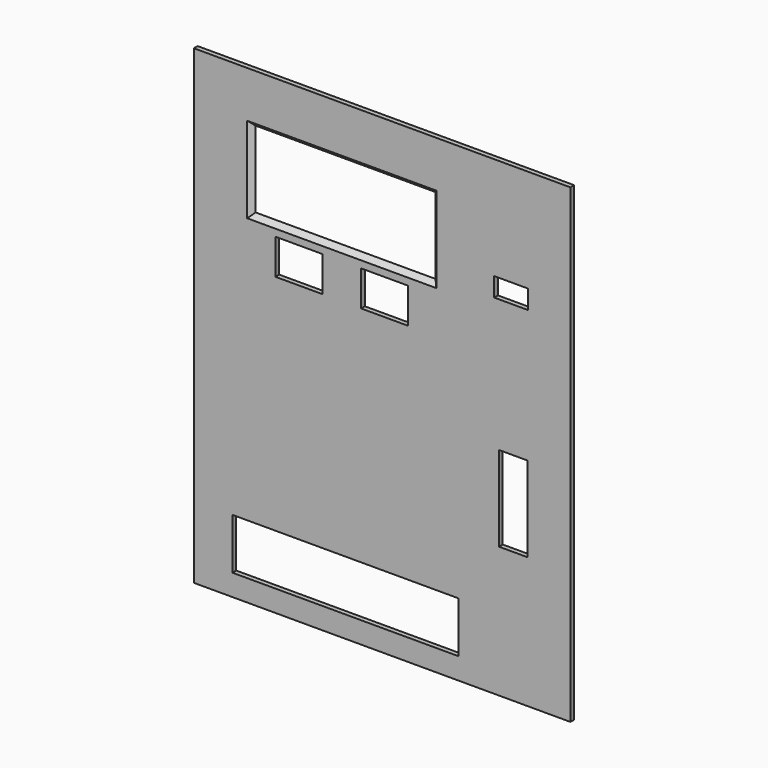
from build123d import *

# Parameters (mm, degrees)
F0_W     = 406.4
F0_H     = 508
F0_W_2   = 244.0329119563
F0_H_2   = 54.9797415733
F0_W_3   = 30.9118032455
F0_H_3   = 91.8955244124
F0_W_4   = 50.8
F0_H_4   = 38.1
F0_W_5   = 194.1293792814
F0_H_5   = 82.4762731791
F0_W_6   = 36.3956689835
F0_H_6   = 20.4090550542
F1_DEPTH = 5.08
F2_SIZE  = 5.07999


# Not quite as in the source:
# - a fillet or chamfer is up to 0.001 mm smaller than in the source, because OpenCascade refuses the exact size


with BuildPart() as f1:
    # F0 (on Front) → F1 (new body)
    with BuildSketch(Plane.XZ):
        with Locations((0.8964706212, 86.9385877169)):
            Rectangle(F0_W, F0_H)
        with Locations((-38.650367409, -116.3898707867)):
            Rectangle(F0_W_2, F0_H_2, mode=Mode.SUBTRACT)
        with Locations((142.4559016228, 20.3487034887)):
            Rectangle(F0_W_3, F0_H_3, mode=Mode.SUBTRACT)
        with Locations((-88.9, 171.45)):
            Rectangle(F0_W_4, F0_H_4, mode=Mode.SUBTRACT)
        with Locations((-42.6353103593, 244.4381365895)):
            Rectangle(F0_W_5, F0_H_5, mode=Mode.SUBTRACT)
        with Locations((3.6293792814, 171.45)):
            Rectangle(F0_W_4, F0_H_4, mode=Mode.SUBTRACT)
        with Locations((140.1178344917, 219.6642868221)):
            Rectangle(F0_W_6, F0_H_6, mode=Mode.SUBTRACT)
    extrude(amount=F1_DEPTH)

    # F2 (size 5.08 in the source; OpenCascade refuses exactly that, so slightly less here)
    f2_edges = [f1.edges().sort_by_distance(p)[0] for p in [
        (-139.7, -5.08, 244.438137),
        (-42.63531, -5.08, 285.676273),
        (54.429379, -5.08, 244.438137),
        (-42.63531, -5.08, 203.2),
    ]]
    chamfer(f2_edges, length=F2_SIZE)


solid = f1.part
